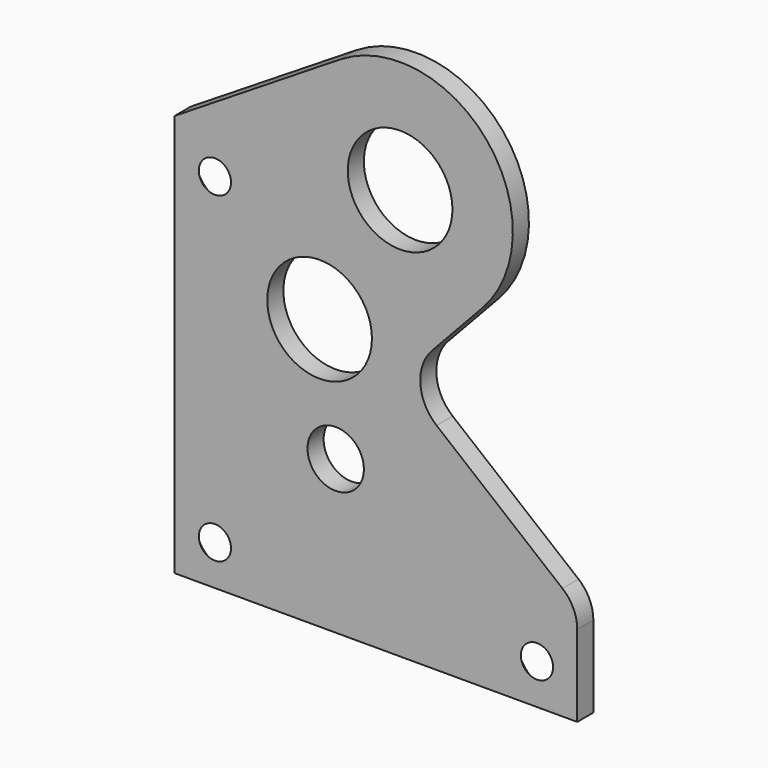
from build123d import *

# Parameters (mm, degrees)
F0_R     = 4
F0_R_2   = 7
F0_R_3   = 13
F1_DEPTH = 5
F2_SIZE  = 4.99999
F3_R     = 10


# Not quite as in the source:
# - a fillet or chamfer is up to 0.001 mm smaller than in the source, because OpenCascade refuses the exact size


with BuildPart() as f1:
    # F0 (on Front) → F1 (new body)
    with BuildSketch(Plane.XZ):
        with BuildLine():
            Line((0, 100), (0, 0))
            Line((0, 0), (100, 0))
            Line((100, 0), (100, 25))
            Line((100, 25), (65.0521931045, 53.4719299169))
            ThreePointArc((65.0521931045, 53.4719299169), (61.0252955601, 61.2544381602), (63.9626496251, 69.51005985))
            Line((63.9626496251, 69.51005985), (76.4587100452, 82.8834840181))
            ThreePointArc((76.4587100452, 82.8834840181), (77.6106511533, 119.803925318), (41.1521770426, 125.7390428077))
            Line((41.1521770426, 125.7390428077), (0, 100))
        make_face()
        with Locations((10, 10)):
            Circle(F0_R, mode=Mode.SUBTRACT)
        with Locations((40, 38)):
            Circle(F0_R_2, mode=Mode.SUBTRACT)
        with Locations((90, 10)):
            Circle(F0_R, mode=Mode.SUBTRACT)
        with Locations((10, 90)):
            Circle(F0_R, mode=Mode.SUBTRACT)
        with Locations((36, 67.24)):
            Circle(F0_R_3, mode=Mode.SUBTRACT)
        with Locations((56, 102)):
            Circle(F0_R_3, mode=Mode.SUBTRACT)
    extrude(amount=F1_DEPTH)

    # F2 (size 5 in the source; OpenCascade refuses exactly that, so slightly less here)
    f2_edges = [f1.edges().sort_by_distance(p)[0] for p in [
        (86, 0, 10),
        (6, 0, 10),
        (6, 0, 90),
    ]]
    chamfer(f2_edges, length=F2_SIZE)

    # F3
    f3_edges = [f1.edges().sort_by_distance(p)[0] for p in [
        (100, -2.5, 25),
    ]]
    fillet(f3_edges, radius=F3_R)


solid = f1.part
